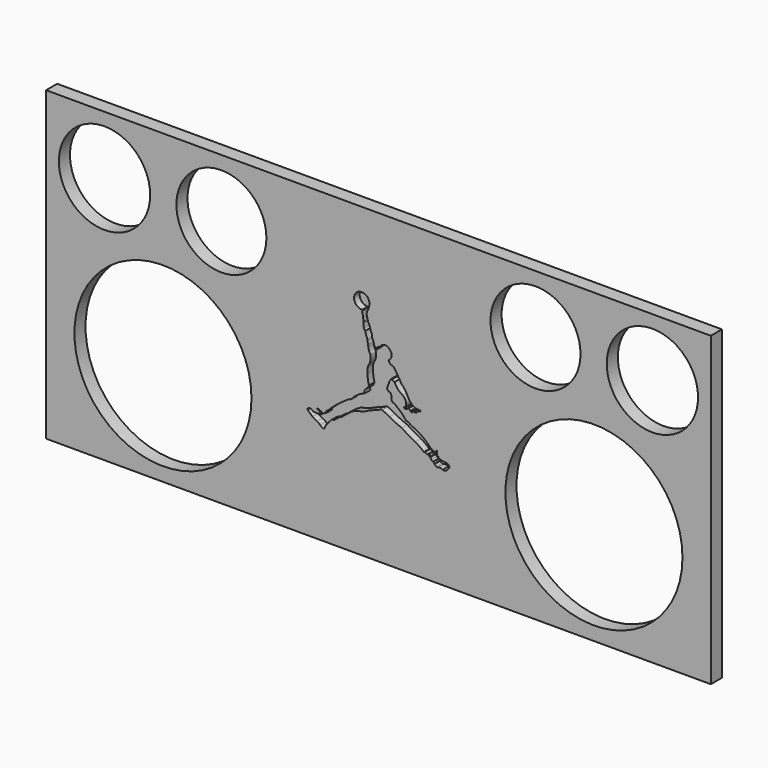
from build123d import *

# Parameters (mm, degrees)
F0_W     = 577.85
F0_H     = 266.7
F0_R     = 76.962
F0_R_2   = 39.6875
F0_R_3   = 39.116
F2_DEPTH = 12.065
F4_DEPTH = 6.0325


# Not quite as in the source:
# - a variable given as a bare number and used for a length is read in inches; the dataset says mm whatever the document's units were
# - ends of sketch curves that miss each other by under 0.0002 mm in the source are joined


with BuildPart() as f2:
    # F0 (on Front) → F2 (new body)
    with BuildSketch(Plane.XZ):
        Rectangle(F0_W, F0_H)
        with Locations((-187.325, -44.45)):
            Circle(F0_R, mode=Mode.SUBTRACT)
        with Locations((187.325, -44.45)):
            Circle(F0_R, mode=Mode.SUBTRACT)
        with Locations((-238.125, 82.55)):
            Circle(F0_R_2, mode=Mode.SUBTRACT)
        with Locations((-136.525, 82.55)):
            Circle(F0_R_3, mode=Mode.SUBTRACT)
        with Locations((136.525, 82.55)):
            Circle(F0_R_3, mode=Mode.SUBTRACT)
        with Locations((238.125, 82.55)):
            Circle(F0_R_2, mode=Mode.SUBTRACT)
    extrude(amount=F2_DEPTH)

    # F3 (on face) → F4 (cut)
    with BuildSketch(Plane.XZ.offset(12.065)):
        with BuildLine():
            ThreePointArc((46.783626309, -33.6210064446), (46.4485261783, -33.282761325), (46.0180841092, -33.0792386392))
            ThreePointArc((46.0180841092, -33.0792386392), (45.9229433317, -32.9007051754), (46.088747805, -32.7848002114))
            ThreePointArc((46.088747805, -32.7848002114), (46.2563523064, -32.4935969953), (46.1005264308, -32.1959242914))
            ThreePointArc((46.1005264308, -32.1959242914), (44.6851106555, -31.093489267), (43.4741346406, -29.7697441665))
            ThreePointArc((43.4741346406, -29.7697441665), (36.3621252426, -24.018722112), (28.167718726, -19.9558871148))
            ThreePointArc((28.167718726, -19.9558871148), (26.3180584023, -18.4009781215), (23.9696554595, -17.8317845402))
            ThreePointArc((23.9696554595, -17.8317845402), (20.1734377128, -13.2259526665), (15.5160421252, -9.4931775731))
            ThreePointArc((15.5160421252, -9.4931775731), (14.5613314413, -8.3666168885), (13.177778956, -7.8504823509))
            ThreePointArc((13.177778956, -7.8504823509), (12.4914927599, -7.5703661305), (11.9300948848, -7.0863348444))
            ThreePointArc((11.9300948848, -7.0863348444), (11.4059776523, -5.9636435072), (11.2823324712, -4.7308234727))
            ThreePointArc((11.2823324712, -4.7308234727), (11.317947086, -3.7872647074), (11.2381630439, -2.8464108763))
            ThreePointArc((11.2381630439, -2.8464108763), (10.9417386094, -1.8674659254), (10.4137326337, -0.9914464005))
            ThreePointArc((10.4137326337, -0.9914464005), (9.6607814879, -0.5010664347), (8.7648788058, -0.4320122508))
            ThreePointArc((8.7648788058, -0.4320122508), (8.1804421328, 0.42892383), (7.4840663371, 1.202125381))
            ThreePointArc((7.4840663371, 1.202125381), (7.9459717223, 2.9707208925), (8.2413290635, 4.7746189622))
            ThreePointArc((8.2413290635, 4.7746189622), (9.1130356749, 5.811599592), (9.1758502106, 7.1648385118))
            ThreePointArc((9.1758502106, 7.1648385118), (10.1961734055, 8.4906531205), (11.0448439891, 9.9323913385))
            ThreePointArc((11.0448439891, 9.9323913385), (11.5182752742, 10.0838607904), (12.0152866026, 10.0761605456))
            ThreePointArc((12.0152866026, 10.0761605456), (12.7005740995, 8.8969740928), (13.9921098528, 8.4587583308))
            ThreePointArc((13.9921098528, 8.4587583308), (16.9074390599, 3.9333156294), (21.1805567276, 0.6592897442))
            ThreePointArc((21.1805567276, 0.6592897442), (23.303001452, -1.8181665265), (24.0918775068, -4.9836424105))
            ThreePointArc((24.0918775068, -4.9836424105), (24.0559917507, -5.3290329727), (23.9800317235, -5.6678728075))
            ThreePointArc((23.9800317235, -5.6678728075), (23.9863795237, -6.0872628989), (24.0918796186, -6.493215076))
            ThreePointArc((24.0918796186, -6.493215076), (24.1380817033, -6.7439220854), (24.0830873569, -6.9928477551))
            ThreePointArc((24.0830873569, -6.9928477551), (23.7405609896, -7.3507541548), (23.2898999953, -7.5564873953))
            ThreePointArc((23.2898999953, -7.5564873953), (22.8598366927, -7.6989293861), (22.4745009503, -7.9371741426))
            ThreePointArc((22.4745009503, -7.9371741426), (22.3787361341, -8.3923019746), (22.5951030897, -8.8040020273))
            ThreePointArc((22.5951030897, -8.8040020273), (23.4684637305, -9.045305888), (24.3513722705, -8.8416919032))
            ThreePointArc((24.3513722705, -8.8416919032), (25.1943230822, -8.363602797), (25.8588969841, -7.6582828726))
            ThreePointArc((25.8588969841, -7.6582828726), (26.1588726672, -7.5562355557), (26.4468346553, -7.6884339093))
            Line((26.4468346553, -7.6884339093), (27.6528579858, -9.1281260859))
            ThreePointArc((27.6528579858, -9.1281260859), (28.034268369, -9.4466709616), (28.4518495908, -9.7160600724))
            ThreePointArc((28.4518495908, -9.7160600724), (28.776662191, -9.8356838582), (29.1226978321, -9.8442015476))
            ThreePointArc((29.1226978321, -9.8442015476), (29.4746754677, -9.6010917515), (29.4694282107, -9.1733518257))
            ThreePointArc((29.4694282107, -9.1733518257), (29.2399037876, -8.7494731194), (28.9568685432, -8.359286424))
            ThreePointArc((28.9568685432, -8.359286424), (28.9501711797, -8.1660125863), (29.1302351728, -8.0954688277))
            ThreePointArc((29.1302351728, -8.0954688277), (29.7826574023, -8.2292210082), (30.3965576175, -8.4874275933))
            ThreePointArc((30.3965576175, -8.4874275933), (31.0806875159, -8.8019380497), (31.8183412572, -8.952993381))
            ThreePointArc((31.8183412572, -8.952993381), (32.428741618, -8.973588861), (33.0319015295, -8.8776158389))
            ThreePointArc((33.0319015295, -8.8776158389), (33.2886882396, -8.6903394602), (33.2957162436, -8.372593868))
            ThreePointArc((33.2957162436, -8.372593868), (32.9174289351, -8.0537302747), (32.4590389341, -7.8675729433))
            ThreePointArc((32.4590389341, -7.8675729433), (31.7525526675, -7.5962447153), (31.1098030658, -7.1967261594))
            ThreePointArc((31.1098030658, -7.1967261594), (31.106411733, -7.0148354866), (31.2775029644, -6.9530082267))
            ThreePointArc((31.2775029644, -6.9530082267), (33.7113261551, -7.2012039327), (36.148698468, -6.990697844))
            ThreePointArc((36.148698468, -6.990697844), (36.4529820354, -6.8549917613), (36.5821110349, -6.5478601425))
            ThreePointArc((36.5821110349, -6.5478601425), (36.5353592164, -6.3060438798), (36.3701376131, -6.1233890544))
            ThreePointArc((36.3701376131, -6.1233890544), (34.3546710667, -5.9663614956), (32.3591516574, -5.6428388328))
            ThreePointArc((32.3591516574, -5.6428388328), (30.9154612592, -5.0643311086), (29.6032033927, -4.2295307309))
            ThreePointArc((29.6032033927, -4.2295307309), (29.2750324862, -3.8121442676), (28.9083205599, -3.428178432))
            ThreePointArc((28.9083205599, -3.428178432), (27.6252990934, -2.2636028661), (26.5228219712, -0.926843875))
            ThreePointArc((26.5228219712, -0.926843875), (23.5422681836, 4.6879483339), (19.5363317213, 9.623742256))
            ThreePointArc((19.5363317213, 9.623742256), (18.5468057965, 11.8690483347), (17.0328816358, 13.8000047576))
            ThreePointArc((17.0328816358, 13.8000047576), (15.7316204623, 16.2684898581), (14.1709334156, 18.5817032251))
            ThreePointArc((14.1709334156, 18.5817032251), (13.5599181013, 19.3841077786), (12.8165122731, 20.0656800028))
            ThreePointArc((12.8165122731, 20.0656800028), (12.0333453581, 20.4505474215), (11.1676539832, 20.5603248428))
            ThreePointArc((11.1676539832, 20.5603248428), (10.1396715718, 21.2902749166), (9.3892432404, 22.3034031882))
            ThreePointArc((9.3892432404, 22.3034031882), (9.1895879777, 22.9774242853), (8.8555700814, 23.5959702726))
            ThreePointArc((8.8555700814, 23.5959702726), (10.4588964493, 25.0491993904), (11.4319106709, 26.9820136883))
            ThreePointArc((11.4319106709, 26.9820136883), (11.5296258271, 28.402200565), (11.2478843414, 29.7975858097))
            ThreePointArc((11.2478843414, 29.7975858097), (9.5278310308, 32.3648406945), (6.8681062796, 33.9381322967))
            ThreePointArc((6.8681062796, 33.9381322967), (4.8679130591, 33.9926959781), (3.0220001951, 33.220453949))
            ThreePointArc((3.0220001951, 33.220453949), (2.3514812012, 32.4923868724), (1.6234156906, 31.8218664803))
            ThreePointArc((1.6234156906, 31.8218664803), (1.1816801821, 31.5840379842), (0.8873194999, 31.1777816044))
            ThreePointArc((0.8873194999, 31.1777816044), (0.2542866736, 31.0364016871), (-0.3566188003, 30.8184251756))
            ThreePointArc((-0.3566188003, 30.8184251756), (-0.5819960596, 30.6668003554), (-0.7246676441, 30.4356520047))
            ThreePointArc((-0.7246676441, 30.4356520047), (-0.7707508187, 29.9766548587), (-0.6952892279, 29.5215642061))
            ThreePointArc((-0.6952892279, 29.5215642061), (-1.1785274301, 29.0067488948), (-1.4141453799, 28.3411372547))
            ThreePointArc((-1.4141453799, 28.3411372547), (-2.3004151276, 29.7233881487), (-3.5994340868, 30.7277007348))
            ThreePointArc((-3.5994340868, 30.7277007348), (-3.6813745105, 30.9308280659), (-3.771958163, 31.1302485556))
            ThreePointArc((-3.771958163, 31.1302485556), (-4.5774191597, 34.0078513128), (-5.7272150594, 36.7659906268))
            ThreePointArc((-5.7272150594, 36.7659906268), (-5.6727203013, 37.9503609491), (-5.8422288134, 39.1238041698))
            ThreePointArc((-5.8422288134, 39.1238041698), (-6.409256895, 40.2981018401), (-7.0671327137, 41.4240216615))
            ThreePointArc((-7.0671327137, 41.4240216615), (-6.9483204957, 41.5893677859), (-6.9291113742, 41.7920680246))
            Line((-6.9291113742, 41.7920680246), (-8.2862919331, 46.2776593465))
            ThreePointArc((-8.2862919331, 46.2776593465), (-8.5175196511, 46.6537215304), (-8.9319015859, 46.8059585289))
            Line((-8.9319015859, 46.8059585289), (-10.3920755007, 52.7240489141))
            ThreePointArc((-10.3920755007, 52.7240489141), (-10.0599210909, 53.7722704264), (-9.8866352382, 54.8581190852))
            ThreePointArc((-9.8866352382, 54.8581190852), (-8.7300093479, 57.0314815841), (-8.1340783047, 59.4202373096))
            ThreePointArc((-8.1340783047, 59.4202373096), (-18.5565652434, 66.7237958013), (-14.2698008884, 54.7407283165))
            ThreePointArc((-14.2698008884, 54.7407283165), (-13.7823939383, 54.3086365266), (-13.9525901035, 53.6799068541))
            ThreePointArc((-13.9525901035, 53.6799068541), (-14.1056995864, 52.9332762142), (-13.9076604603, 52.1972880927))
            ThreePointArc((-13.9076604603, 52.1972880927), (-13.5401617408, 50.6269798419), (-13.3325976574, 49.0276554119))
            Line((-13.3325976574, 49.0276554119), (-12.9731720142, 45.5771994276))
            ThreePointArc((-12.9731720142, 45.5771994276), (-13.1128496352, 45.2511506342), (-13.1399340307, 44.8974782022))
            ThreePointArc((-13.1399340307, 44.8974782022), (-12.9964146938, 43.1447939246), (-12.6338670604, 41.4240210428))
            ThreePointArc((-12.6338670604, 41.4240210428), (-12.255479415, 40.301346049), (-11.4607100679, 39.422757846))
            ThreePointArc((-11.4607100679, 39.422757846), (-10.7012757005, 36.3969845177), (-9.5744657125, 33.4879756095))
            ThreePointArc((-9.5744657125, 33.4879756095), (-9.4489695101, 31.6730739053), (-8.8613751833, 29.9513443346))
            ThreePointArc((-8.8613751833, 29.9513443346), (-8.8818695461, 28.8469890124), (-8.8337180617, 27.7434954992))
            ThreePointArc((-8.8337180617, 27.7434954992), (-8.6178847127, 26.5791766285), (-8.2264372409, 25.4615938857))
            ThreePointArc((-8.2264372409, 25.4615938857), (-7.6926556539, 24.0535488761), (-7.0302786624, 22.7012285571))
            ThreePointArc((-7.0302786624, 22.7012285571), (-6.8748174454, 22.2478408566), (-6.8094485821, 21.773019568))
            ThreePointArc((-6.8094485821, 21.773019568), (-6.7657072034, 20.6953748679), (-6.809447602, 19.6177301774))
            ThreePointArc((-6.809447602, 19.6177301774), (-7.0454506417, 18.0564445921), (-7.4336682743, 16.5258898463))
            ThreePointArc((-7.4336682743, 16.5258898463), (-7.8648831959, 15.3765952803), (-8.4610937297, 14.3035821822))
            ThreePointArc((-8.4610937297, 14.3035821822), (-9.037657541, 13.2184813217), (-9.3352084245, 12.0262844426))
            ThreePointArc((-9.3352084245, 12.0262844426), (-9.5116313904, 9.7683798359), (-9.5583635565, 7.5040753585))
            ThreePointArc((-9.5583635565, 7.5040753585), (-9.2047430334, 3.0463568939), (-8.2806149218, -1.3288330427))
            ThreePointArc((-8.2806149218, -1.3288330427), (-8.8254046738, -2.4979404008), (-9.2283249076, -3.7232012339))
            ThreePointArc((-9.2283249076, -3.7232012339), (-10.6555228217, -4.5904844372), (-11.8598698233, -5.7474744262))
            ThreePointArc((-11.8598698233, -5.7474744262), (-12.2013903174, -6.6085211705), (-12.1359059284, -7.5325074294))
            ThreePointArc((-12.1359059284, -7.5325074294), (-11.8974981667, -7.952575725), (-11.6390414547, -8.3606154127))
            ThreePointArc((-11.6390414547, -8.3606154127), (-18.3595100529, -11.9707379825), (-23.9801787386, -17.1288110633))
            ThreePointArc((-23.9801787386, -17.1288110633), (-25.316910356, -17.4273386554), (-26.5364187889, -18.0508504351))
            ThreePointArc((-26.5364187889, -18.0508504351), (-34.8440391846, -24.0153621053), (-42.5910653341, -30.6918540233))
            ThreePointArc((-42.5910653341, -30.6918540233), (-43.6089502096, -31.705065949), (-44.7777679351, -32.5396636437))
            ThreePointArc((-44.7777679351, -32.5396636437), (-44.9632966605, -32.6286656372), (-45.1458148436, -32.7236884589))
            ThreePointArc((-45.1458148436, -32.7236884589), (-45.4169832298, -33.0754879333), (-45.3068348214, -33.5057917755))
            ThreePointArc((-45.3068348214, -33.5057917755), (-45.1848490319, -33.7610895542), (-45.0538042886, -34.0118572405))
            ThreePointArc((-45.0538042886, -34.0118572405), (-45.3275510704, -34.4810331427), (-45.8129044363, -34.7249501548))
            ThreePointArc((-45.8129044363, -34.7249501548), (-46.2767397833, -34.6724666205), (-46.7330257173, -34.7709609998))
            ThreePointArc((-46.7330257173, -34.7709609998), (-47.1719928987, -35.1653733975), (-47.653146386, -35.5070526379))
            ThreePointArc((-47.653146386, -35.5070526379), (-48.1675931816, -35.6414020172), (-48.6763246862, -35.4868107755))
            ThreePointArc((-48.6763246862, -35.4868107755), (-49.0095300916, -35.2327484401), (-49.2799255163, -34.9126548735))
            ThreePointArc((-49.2799255163, -34.9126548735), (-49.6111686088, -34.8709814643), (-49.9424113652, -34.9126573765))
            ThreePointArc((-49.9424113652, -34.9126573765), (-51.0800303379, -33.9447888166), (-52.5187512142, -33.5435153879))
            ThreePointArc((-52.5187512142, -33.5435153879), (-52.7684767989, -33.5194686929), (-53.0192993797, -33.514074811))
            ThreePointArc((-53.0192993797, -33.514074811), (-53.2602922841, -33.7669222264), (-53.0929083746, -34.0735047793))
            ThreePointArc((-53.0929083746, -34.0735047793), (-52.5710510057, -34.2190277661), (-52.0770944347, -34.441555386))
            ThreePointArc((-52.0770944347, -34.441555386), (-50.7006041581, -35.5628008537), (-49.662694155, -37.0031695905))
            Line((-49.662694155, -37.0031695905), (-55.9783856899, -37.1903138157))
            ThreePointArc((-55.9783856899, -37.1903138157), (-56.5238459404, -36.9877186598), (-57.0236429091, -36.6897679104))
            ThreePointArc((-57.0236429091, -36.6897679104), (-57.9124942767, -36.0661234051), (-58.8933307479, -35.6003455471))
            ThreePointArc((-58.8933307479, -35.6003455471), (-59.5897327593, -35.4868805264), (-60.2919056555, -35.5561838444))
            ThreePointArc((-60.2919056555, -35.5561838444), (-60.996643883, -35.8387699564), (-61.5285484543, -36.3806086535))
            ThreePointArc((-61.5285484543, -36.3806086535), (-61.6425037867, -36.7493913551), (-61.5874372961, -37.1314306274))
            ThreePointArc((-61.5874372961, -37.1314306274), (-59.4812175794, -39.2363235447), (-57.2002966032, -41.1505161363))
            ThreePointArc((-57.2002966032, -41.1505161363), (-55.4260457929, -42.4324566212), (-53.495890989, -43.4648515116))
            ThreePointArc((-53.495890989, -43.4648515116), (-51.9248853494, -44.309976728), (-50.5284995544, -45.4201125272))
            ThreePointArc((-50.5284995544, -45.4201125272), (-49.4696547302, -46.4236079708), (-48.228969331, -47.1909770212))
            ThreePointArc((-48.228969331, -47.1909770212), (-47.7358683452, -47.2672140848), (-47.2850736744, -47.0533336519))
            ThreePointArc((-47.2850736744, -47.0533336519), (-46.4303651048, -45.6883643859), (-45.8128796093, -44.2009576656))
            ThreePointArc((-45.8128796093, -44.2009576656), (-45.7537500994, -43.9629437192), (-45.7438697383, -43.7178940617))
            ThreePointArc((-45.7438697383, -43.7178940617), (-44.4781220767, -42.4966581291), (-43.5125754812, -41.0265366894))
            ThreePointArc((-43.5125754812, -41.0265366894), (-42.3263705098, -40.0607178539), (-41.3732921572, -38.8642533052))
            ThreePointArc((-41.3732921572, -38.8642533052), (-40.7814232976, -38.2306943546), (-40.085121604, -37.7140997575))
            ThreePointArc((-40.085121604, -37.7140997575), (-39.1907342799, -37.6752302358), (-38.3341423196, -37.4150580883))
            ThreePointArc((-38.3341423196, -37.4150580883), (-35.8237711209, -35.5707866071), (-33.4464549703, -33.5579103978))
            ThreePointArc((-33.4464549703, -33.5579103978), (-32.3768465639, -33.282110003), (-31.4095147087, -32.7488219956))
            ThreePointArc((-31.4095147087, -32.7488219956), (-28.5580047918, -30.2626473992), (-25.5391422224, -27.9825943826))
            ThreePointArc((-25.5391422224, -27.9825943826), (-24.3347071434, -27.0251166982), (-23.0399130435, -26.1938914343))
            ThreePointArc((-23.0399130435, -26.1938914343), (-21.763478679, -25.5513313188), (-20.5958389315, -24.7274469433))
            ThreePointArc((-20.5958389315, -24.7274469433), (-18.6822322552, -24.1877915225), (-16.7428269569, -23.7498123832))
            ThreePointArc((-16.7428269569, -23.7498123832), (-13.417396887, -22.9447682367), (-10.2803982434, -21.5788175499))
            ThreePointArc((-10.2803982434, -21.5788175499), (-9.3684361196, -21.0826635825), (-8.4114014009, -20.6802602942))
            ThreePointArc((-8.4114014009, -20.6802602942), (-6.1930661166, -19.7873135828), (-4.0264462369, -18.7753234753))
            ThreePointArc((-4.0264462369, -18.7753234753), (-1.0076469353, -17.7625699294), (1.8590803463, -16.3766774289))
            ThreePointArc((1.8590803463, -16.3766774289), (2.5654878307, -16.2661712096), (3.2518392647, -16.4665340702))
            ThreePointArc((3.2518392647, -16.4665340702), (6.5092027352, -17.8776545765), (9.631593359, -19.5665460902))
            ThreePointArc((9.631593359, -19.5665460902), (14.8160322838, -22.2827505387), (20.2180177864, -24.5354656487))
            ThreePointArc((20.2180177864, -24.5354656487), (26.0473977942, -28.1781249391), (32.113465613, -31.4113050866))
            ThreePointArc((32.113465613, -31.4113050866), (35.7808132881, -33.7900500502), (39.1941026422, -36.5208595998))
            ThreePointArc((39.1941026422, -36.5208595998), (39.5311966368, -36.6555865836), (39.8913820076, -36.6103103468))
            ThreePointArc((39.8913820076, -36.6103103468), (40.0921702775, -36.5192692028), (40.2824317515, -36.407891473))
            ThreePointArc((40.2824317515, -36.407891473), (40.4958619415, -36.3616153514), (40.6946450352, -36.4520568601))
            ThreePointArc((40.6946450352, -36.4520568601), (41.3033027779, -36.935457384), (41.9607328265, -37.3500971182))
            ThreePointArc((41.9607328265, -37.3500971182), (42.3808384199, -37.4582220089), (42.8146053687, -37.4531487415))
            ThreePointArc((42.8146053687, -37.4531487415), (43.18508202, -37.7318148772), (43.6243126982, -37.880085566))
            ThreePointArc((43.6243126982, -37.880085566), (44.1120974855, -38.2920339016), (44.4192972343, -38.8517339487))
            ThreePointArc((44.4192972343, -38.8517339487), (44.6669587913, -38.9920630259), (44.9492866867, -39.0283963174))
            ThreePointArc((44.9492866867, -39.0283963174), (45.517335964, -39.6761746137), (45.9650950773, -40.4122519894))
            ThreePointArc((45.9650950773, -40.4122519894), (46.3901741804, -41.0069237421), (47.0250752181, -41.3691767397))
            ThreePointArc((47.0250752181, -41.3691767397), (47.2862118988, -41.433346679), (47.5550653038, -41.4280640742))
            ThreePointArc((47.5550653038, -41.4280640742), (47.9881263474, -41.8402100474), (48.291160291, -42.3555483435))
            ThreePointArc((48.291160291, -42.3555483435), (48.4626373148, -42.697726503), (48.8358741768, -42.7824828884))
            ThreePointArc((48.8358741768, -42.7824828884), (48.9593970877, -43.1685566046), (49.2098176277, -43.4873030632))
            ThreePointArc((49.2098176277, -43.4873030632), (49.6618743517, -43.924908281), (50.1755769198, -44.288175556))
            ThreePointArc((50.1755769198, -44.288175556), (50.640003601, -44.4460047289), (51.1295596384, -44.476618887))
            ThreePointArc((51.1295596384, -44.476618887), (51.4826920946, -44.4941263304), (51.8362117268, -44.4883965059))
            ThreePointArc((51.8362117268, -44.4883965059), (53.34334921, -44.1614453193), (54.8394915739, -44.5355044224))
            ThreePointArc((54.8394915739, -44.5355044224), (55.3813786166, -44.8088240903), (55.8806118615, -45.1539491889))
            ThreePointArc((55.8806118615, -45.1539491889), (57.0229427332, -45.2374150693), (58.1513310681, -45.040883147))
            ThreePointArc((58.1513310681, -45.040883147), (59.1834892717, -44.4532340926), (60.0727965872, -43.6659510222))
            ThreePointArc((60.0727965872, -43.6659510222), (60.8895244728, -42.6463757381), (61.5621088695, -41.5264612479))
            ThreePointArc((61.5621088695, -41.5264612479), (61.6427796678, -40.9962899686), (61.5338424717, -40.4711974916))
            ThreePointArc((61.5338424717, -40.4711974916), (60.742886265, -39.6242595583), (59.7907639218, -38.9636699506))
            ThreePointArc((59.7907639218, -38.9636699506), (58.6551282529, -38.6595849858), (57.4823639814, -38.577366457))
            Line((57.4823639814, -38.577366457), (56.5118917696, -38.5585225724))
            ThreePointArc((56.5118917696, -38.5585225724), (55.3267983453, -38.2470640795), (54.2152620208, -37.7313707149))
            Line((54.2152620208, -37.7313707149), (53.5086060669, -37.7313715724))
            ThreePointArc((53.5086060669, -37.7313715724), (52.8671068614, -37.3780166018), (52.1777419099, -37.1307174684))
            ThreePointArc((52.1777419099, -37.1307174684), (52.185150475, -36.7518985169), (52.1306310729, -36.3769511194))
            ThreePointArc((52.1306310729, -36.3769511194), (51.8312120036, -35.9710853636), (51.38864633, -35.7291864492))
            ThreePointArc((51.38864633, -35.7291864492), (51.0819465913, -35.6936272934), (50.7879932122, -35.788075502))
            ThreePointArc((50.7879932122, -35.788075502), (50.5134750657, -35.7675694812), (50.5406639818, -35.4936348308))
            ThreePointArc((50.5406639818, -35.4936348308), (50.7791034386, -34.9214473439), (50.8351049205, -34.3041013136))
            ThreePointArc((50.8351049205, -34.3041013136), (50.8514404191, -33.9436820745), (50.9528770675, -33.5974453759))
            ThreePointArc((50.9528770675, -33.5974453759), (51.0964790432, -33.1008614211), (51.0706550137, -32.584575839))
            ThreePointArc((51.0706550137, -32.584575839), (50.923957305, -32.3060813989), (50.6584368209, -32.13703134))
            ThreePointArc((50.6584368209, -32.13703134), (50.3588114124, -32.2568300716), (50.1637808927, -32.5139120975))
            ThreePointArc((50.1637808927, -32.5139120975), (49.9411440458, -33.2182586693), (49.8457853754, -33.9507736491))
            ThreePointArc((49.8457853754, -33.9507736491), (49.7965652689, -34.2608081408), (49.5984592639, -34.5043205057))
            ThreePointArc((49.5984592639, -34.5043205057), (49.2643121463, -34.6150220923), (48.9389152611, -34.4807628502))
            ThreePointArc((48.9389152611, -34.4807628502), (48.7421950093, -34.182855279), (48.5973659686, -33.8565543893))
            ThreePointArc((48.5973659686, -33.8565543893), (48.398572861, -33.4265225707), (48.0320461615, -33.1263495296))
            ThreePointArc((48.0320461615, -33.1263495296), (47.6329824763, -33.0694698269), (47.2547278729, -33.2087916881))
            ThreePointArc((47.2547278729, -33.2087916881), (46.9964427833, -33.3889168999), (46.783626309, -33.6210064446))
        make_face()
    extrude(amount=-F4_DEPTH, mode=Mode.SUBTRACT)


solid = f2.part
